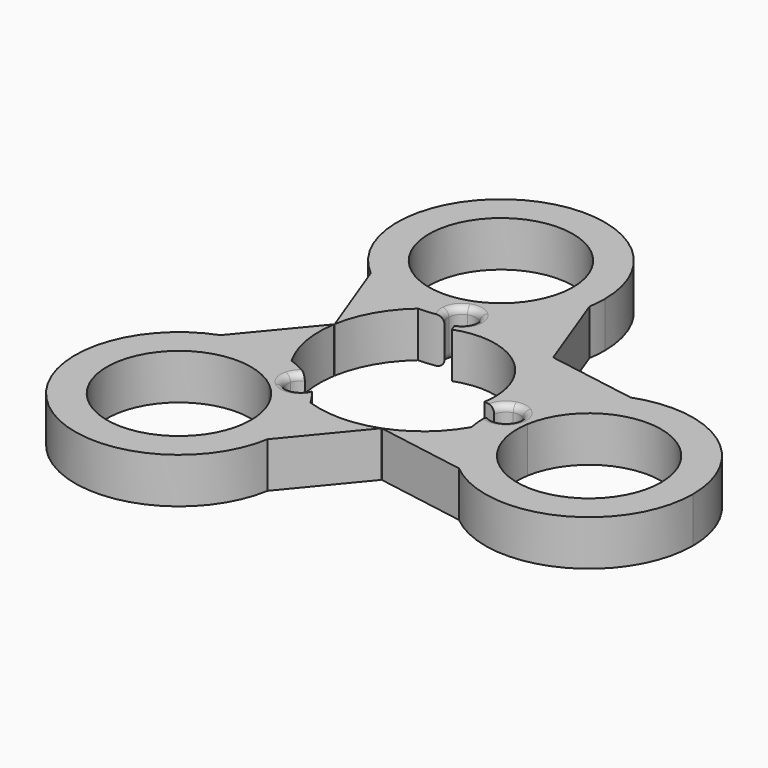
from build123d import *

# Parameters (mm, degrees)
F1_DEPTH = 7
F2_R     = 1
F2_2_R   = 1


# Not quite as in the source:
# - a feature of the source that left no trace in its solid (it failed there, or was rolled back) is left out
# - a feature names something its author has since deleted; it is built from what else it names


with BuildPart() as f1:
    # F0 (on Top) → F1 (new body)
    with BuildSketch(Plane.XY):
        with BuildLine():
            ThreePointArc((-3.8756868885, 10.4013965957), (6.3320563618, 9.1167462524), (11.1, 0))
            ThreePointArc((11.1, 0), (11.0613620354, -0.9253485413), (10.945717131, -1.8442549953))
            Line((10.945717131, -1.8442549953), (12.6838920809, -2.1371218578))
            ThreePointArc((12.6838920809, -2.1371218578), (13.2129796762, -1.0512641279), (14.2462328012, -0.4256375039))
            ThreePointArc((14.2462328012, -0.4256375039), (14.8814025515, 1.3291999624), (15.716588667, 2.998139535))
            ThreePointArc((15.716588667, 2.998139535), (13.7693026548, 8.1490063443), (10.1910345838, 12.3346185232))
            ThreePointArc((10.1910345838, 12.3346185232), (5.4056324272, 15.0591878288), (-0.0200700936, 15.9999874122))
            ThreePointArc((-0.0200700936, 15.9999874122), (-1.5015245737, 14.8650038141), (-3.1050613973, 13.9102447869))
            ThreePointArc((-3.1050613973, 13.9102447869), (-3.5245708313, 12.7775345292), (-4.4911442206, 12.0531336898))
            Line((-4.4911442206, 12.0531336898), (-3.8756868885, 10.4013965957))
        make_face()
        with BuildLine():
            ThreePointArc((-10.4547593349, 12.111895279), (-8.5918222099, 12.2230726724), (-6.7545035094, 12.550418266))
            ThreePointArc((-6.7545035094, 12.550418266), (-7.24022237, 13.309670852), (-7.3697680312, 14.2016379043))
            ThreePointArc((-7.3697680312, 14.2016379043), (-8.9733048548, 13.2468788771), (-10.4547593349, 12.111895279))
        make_face()
        with BuildLine():
            ThreePointArc((-3.1000897142, 14.0559413456), (-3.1013329966, 13.9830506657), (-3.1050613973, 13.9102447869))
            ThreePointArc((-3.1050613973, 13.9102447869), (-1.5015245737, 14.8650038141), (-0.0200700936, 15.9999874122))
            ThreePointArc((-0.0200700936, 15.9999874122), (-1.8830072186, 15.8888100188), (-3.720325919, 15.5614644252))
            ThreePointArc((-3.720325919, 15.5614644252), (-3.2612226734, 14.8700808749), (-3.1000897142, 14.0559413456))
        make_face()
        with BuildLine():
            ThreePointArc((15.716588667, 2.998139535), (14.8814025515, 1.3291999624), (14.2462328012, -0.4256375039))
            ThreePointArc((14.2462328012, -0.4256375039), (15.1466242588, -0.3846189245), (15.9838632161, -0.7184126172))
            ThreePointArc((15.9838632161, -0.7184126172), (15.9959652953, -0.3592969121), (16, 0))
            ThreePointArc((16, 0), (15.9289895893, 1.5057525241), (15.716588667, 2.998139535))
        make_face()
        with BuildLine():
            ThreePointArc((15.3367864718, -4.5588354563), (14.4363950142, -4.5998540357), (13.5991560569, -4.2660603431))
            ThreePointArc((13.5991560569, -4.2660603431), (13.6242332173, -6.1321434818), (13.866430606, -7.9826124952))
            ThreePointArc((13.866430606, -7.9826124952), (14.7016167215, -6.3136729226), (15.3367864718, -4.5588354563))
        make_face()
        with BuildLine():
            ThreePointArc((-15.7691718891, 2.707991494), (-13.9295367407, 7.8719760029), (-10.4547593349, 12.111895279))
            ThreePointArc((-10.4547593349, 12.111895279), (-15.8804618557, 13.0526948625), (-20.6658640122, 15.777264168))
            Line((-20.6658640122, 15.777264168), (-15.7691718891, 2.707991494))
        make_face()
        with BuildLine():
            ThreePointArc((-20.6658640122, 15.777264168), (-15.8804618557, 13.0526948625), (-10.4547593349, 12.111895279))
            ThreePointArc((-10.4547593349, 12.111895279), (-8.9733048548, 13.2468788771), (-7.3697680312, 14.2016379043))
            ThreePointArc((-7.3697680312, 14.2016379043), (-6.9502585972, 15.334348162), (-5.9836852078, 16.0587490014))
            Line((-5.9836852078, 16.0587490014), (-6.5991425399, 17.7104860955))
            ThreePointArc((-6.5991425399, 17.7104860955), (-19.5915756809, 34.443939053), (0.6251705715, 28.1118826912))
            ThreePointArc((0.6251705715, 28.1118826912), (0.5865326069, 27.1865341499), (0.4708877026, 26.2676276959))
            Line((0.4708877026, 26.2676276959), (5.3027808505, 25.4534971124))
            ThreePointArc((5.3027808505, 25.4534971124), (5.4694762081, 26.7780469561), (5.5251705715, 28.1118826912))
            ThreePointArc((5.5251705715, 28.1118826912), (-17.2918466156, 42.5869742857), (-20.6658640122, 15.777264168))
        make_face()
        with BuildLine():
            ThreePointArc((-3.720325919, 15.5614644252), (-1.8830072186, 15.8888100188), (-0.0200700936, 15.9999874122))
            ThreePointArc((-0.0200700936, 15.9999874122), (3.4670684087, 20.2618199719), (5.3027808505, 25.4534971124))
            Line((5.3027808505, 25.4534971124), (0.4708877026, 26.2676276959))
            ThreePointArc((0.4708877026, 26.2676276959), (-1.917687828, 21.0418524487), (-6.5991425399, 17.7104860955))
            Line((-6.5991425399, 17.7104860955), (-5.9836852078, 16.0587490014))
            ThreePointArc((-5.9836852078, 16.0587490014), (-4.7787610312, 16.143474568), (-3.720325919, 15.5614644252))
        make_face()
        with BuildLine():
            ThreePointArc((5.3027808505, 25.4534971124), (3.4670684087, 20.2618199719), (-0.0200700936, 15.9999874122))
            ThreePointArc((-0.0200700936, 15.9999874122), (5.4056324272, 15.0591878288), (10.1910345838, 12.3346185232))
            Line((10.1910345838, 12.3346185232), (5.3027808505, 25.4534971124))
        make_face()
        with BuildLine():
            ThreePointArc((10.1910345838, 12.3346185232), (13.7693026548, 8.1490063443), (15.716588667, 2.998139535))
            ThreePointArc((15.716588667, 2.998139535), (19.2441962666, 7.2265359596), (23.9964435778, 10.0085311417))
            Line((23.9964435778, 10.0085311417), (10.1910345838, 12.3346185232))
        make_face()
        with BuildLine():
            ThreePointArc((23.9964435778, 10.0085311417), (19.2441962666, 7.2265359596), (15.716588667, 2.998139535))
            ThreePointArc((15.716588667, 2.998139535), (15.9289895893, 1.5057525241), (16, 0))
            ThreePointArc((16, 0), (15.9959652953, -0.3592969121), (15.9838632161, -0.7184126172))
            ThreePointArc((15.9838632161, -0.7184126172), (16.6778560085, -1.4873208018), (16.9288346365, -2.4922364801))
            ThreePointArc((16.9288346365, -2.4922364801), (16.9213948268, -2.670414009), (16.8991271921, -2.8473511024))
            ThreePointArc((16.8991271921, -2.8473511024), (16.3700395969, -3.9332088324), (15.3367864718, -4.5588354563))
            ThreePointArc((15.3367864718, -4.5588354563), (14.7016167215, -6.3136729226), (13.866430606, -7.9826124952))
            ThreePointArc((13.866430606, -7.9826124952), (15.8137166182, -13.1334793045), (19.3919846893, -17.3190914834))
            ThreePointArc((19.3919846893, -17.3190914834), (36.4000364602, -19.4595645548), (45.583019273, -4.9844729602))
            ThreePointArc((45.583019273, -4.9844729602), (38.7103077224, 8.1567828991), (23.9964435778, 10.0085311417))
        make_face()
        with BuildLine():
            ThreePointArc((40.683019273, -4.9844729602), (28.6576707318, -16.0458349956), (18.637302142, -3.140217965))
            ThreePointArc((18.637302142, -3.140217965), (30.5083678143, 6.0768890751), (40.683019273, -4.9844729602))
        make_face(mode=Mode.SUBTRACT)
        with BuildLine():
            ThreePointArc((19.3919846893, -17.3190914834), (15.8137166182, -13.1334793045), (13.866430606, -7.9826124952))
            ThreePointArc((13.866430606, -7.9826124952), (10.3580114705, -12.194736503), (5.6336996191, -14.9753607169))
            Line((5.6336996191, -14.9753607169), (19.3919846893, -17.3190914834))
        make_face()
    extrude(amount=F1_DEPTH)

    # F2
    f2_edges = [f1.edges().sort_by_distance(p)[0] for p in [
        (-4.778761, 16.143475, 0),
        (16.755064, -1.648074, 0),
        (16.755064, -1.648074, 7),
        (-4.778761, 16.143475, 7),
    ]]
    fillet(f2_edges, radius=F2_R)


with BuildPart() as f1b:
    # F0 (on Top) → F1, piece 2 (new body)
    with BuildSketch(Plane.XY):
        with BuildLine():
            ThreePointArc((-11.6164605528, -11.0026289688), (-11.2017879557, -10.2023578035), (-10.4940946597, -9.6441844438))
            ThreePointArc((-10.4940946597, -9.6441844438), (-12.1227086435, -8.7328603323), (-13.8463605124, -8.017374917))
            ThreePointArc((-13.8463605124, -8.017374917), (-12.8186095029, -9.5751370962), (-11.6164605528, -11.0026289688))
        make_face()
        with BuildLine():
            ThreePointArc((-5.2618293321, -15.110034814), (-6.2895803416, -13.5522726347), (-7.4917292918, -12.1247807621))
            ThreePointArc((-7.4917292918, -12.1247807621), (-7.9064018888, -12.9250519275), (-8.6140951849, -13.4832252872))
            ThreePointArc((-8.6140951849, -13.4832252872), (-6.985481201, -14.3945493987), (-5.2618293321, -15.110034814))
        make_face()
        with BuildLine():
            ThreePointArc((-11.6164605528, -11.0026289688), (-12.8186095029, -9.5751370962), (-13.8463605124, -8.017374917))
            ThreePointArc((-13.8463605124, -8.017374917), (-19.2807850269, -7.1283406673), (-24.6947655397, -8.134405629))
            ThreePointArc((-24.6947655397, -8.134405629), (-29.2992244283, -35.4620282542), (-3.3305795656, -25.7857953098))
            ThreePointArc((-3.3305795656, -25.7857953098), (-3.163884208, -24.4612454661), (-3.1081898446, -23.127409731))
            ThreePointArc((-3.1081898446, -23.127409731), (-3.6559769254, -18.9766127111), (-5.2618293321, -15.110034814))
            ThreePointArc((-5.2618293321, -15.110034814), (-6.985481201, -14.3945493987), (-8.6140951849, -13.4832252872))
            ThreePointArc((-8.6140951849, -13.4832252872), (-9.8048057602, -13.686274589), (-10.9154419843, -13.2113978989))
            ThreePointArc((-10.9154419843, -13.2113978989), (-11.5912785656, -12.2102657357), (-11.6164605528, -11.0026289688))
        make_face()
        with BuildLine():
            ThreePointArc((-8.0081898446, -23.127409731), (-29.1502846383, -27.8567154046), (-12.0381596021, -14.5702681305))
            ThreePointArc((-12.0381596021, -14.5702681305), (-9.0660950509, -18.3981040574), (-8.0081898446, -23.127409731))
        make_face(mode=Mode.SUBTRACT)
        with BuildLine():
            ThreePointArc((-24.6947655397, -8.134405629), (-19.2807850269, -7.1283406673), (-13.8463605124, -8.017374917))
            ThreePointArc((-13.8463605124, -8.017374917), (-15.7399573393, -2.8729328146), (-15.7858926212, 2.608753371))
            Line((-15.7858926212, 2.608753371), (-24.6947655397, -8.134405629))
        make_face()
        with BuildLine():
            ThreePointArc((5.5865756952, -14.993004102), (0.1725951823, -15.9990690636), (-5.2618293321, -15.110034814))
            ThreePointArc((-5.2618293321, -15.110034814), (-3.6559769254, -18.9766127111), (-3.1081898446, -23.127409731))
            ThreePointArc((-3.1081898446, -23.127409731), (-3.163884208, -24.4612454661), (-3.3305795656, -25.7857953098))
            Line((-3.3305795656, -25.7857953098), (5.5865756952, -14.993004102))
        make_face()
    extrude(amount=F1_DEPTH)

    # F2#2
    f2_2_edges = [f1b.edges().sort_by_distance(p)[0] for p in [
        (-10.915442, -13.211398, 0),
        (-10.915442, -13.211398, 7),
    ]]
    fillet(f2_2_edges, radius=F2_2_R)


solid = Compound([f1.part, f1b.part])
